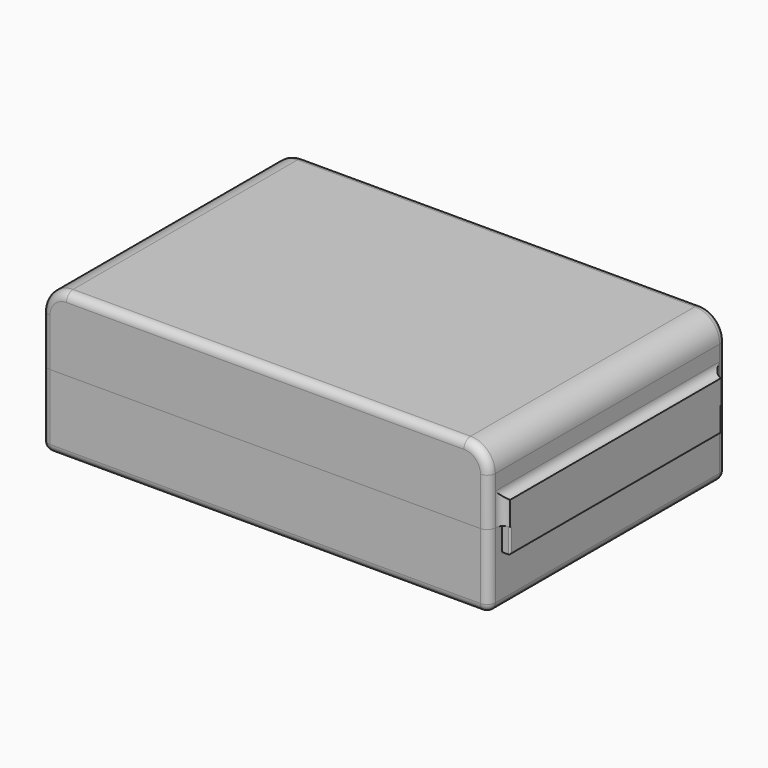
from build123d import *

# Parameters (mm, degrees)
F0_W         = 68.834
F0_H         = 45.72
F1_DEPTH     = 5.08
F2_W         = 68.834
F2_H         = 45.72
F2_W_2       = 58.674
F2_H_2       = 35.56
F3_DEPTH     = 6.35
F4_W         = 68.834
F4_H         = 45.72
F4_W_2       = 58.674
F4_H_2       = 35.56
F5_DEPTH     = 6.35
F6_W         = 68.834
F6_H         = 45.72
F7_DEPTH     = 4.826
F8_W         = 40.64
F8_H         = 3.81
F8_H_2       = 3.683
F9_DEPTH     = 1.27
F10_R        = 3.81
F11_R        = 1.26999
F11_2_R      = 1.26999
F12_T1_DEPTH = 4.4450001001
F12_T3_DEPTH = 41.91


# Not quite as in the source:
# - a fillet or chamfer that OpenCascade refuses, or shapes differently, is made with other operations: its cross-section is extruded or revolved along the edge and cut away or added
# - a fillet or chamfer is up to 0.001 mm smaller than in the source, because OpenCascade refuses the exact size
# - a feature names something its author has since deleted; it is built from what else it names


with BuildPart() as f1:
    # F0 (on Top) → F1 (new body)
    with BuildSketch(Plane.XY):
        with Locations((34.417, 22.86)):
            Rectangle(F0_W, F0_H)
    extrude(amount=F1_DEPTH)

    # F2 (on face) → F3 (join)
    with BuildSketch(Plane.XY.offset(5.08)):
        with Locations((34.417, 22.86)):
            Rectangle(F2_W, F2_H)
        with Locations((34.417, 22.86)):
            Rectangle(F2_W_2, F2_H_2, mode=Mode.SUBTRACT)
    extrude(amount=F3_DEPTH)

    # F11 (radius 1.27 in the source; OpenCascade refuses exactly that, so slightly less here)
    f11_edges = [f1.edges().sort_by_distance(p)[0] for p in [
        (68.834, 0, 5.715),
        (0, 0, 5.715),
        (34.417, 0, 0),
        (68.834, 22.86, 0),
        (68.834, 45.72, 5.715),
        (34.417, 45.72, 0),
        (0, 45.72, 5.715),
        (0, 22.86, 0),
    ]]
    fillet(f11_edges, radius=F11_R)


with BuildPart() as f5:
    # F4 (on face) → F5 (new body)
    with BuildSketch(Plane.XY.offset(11.43)):
        with Locations((34.417, 22.86)):
            Rectangle(F4_W, F4_H)
        with Locations((34.417, 22.86)):
            Rectangle(F4_W_2, F4_H_2, mode=Mode.SUBTRACT)
    extrude(amount=F5_DEPTH)

    # F6 (on face) → F7 (join)
    with BuildSketch(Plane.XY.offset(17.78)):
        with Locations((34.417, 22.86)):
            Rectangle(F6_W, F6_H)
    extrude(amount=F7_DEPTH)

    # F8 (on face) → F9 (join)
    with BuildSketch(Plane.YZ.offset(68.834)):
        with Locations((22.86, 9.525)):
            Rectangle(F8_W, F8_H)
        with Locations((22.86, 13.2715)):
            Rectangle(F8_W, F8_H_2)
    extrude(amount=F9_DEPTH)

    # F10
    f10_edges = [f5.edges().sort_by_distance(p)[0] for p in [
        (68.834, 22.86, 22.606),
        (0, 22.86, 22.606),
    ]]
    fillet(f10_edges, radius=F10_R)

    # F11#2 (radius 1.27 in the source; OpenCascade refuses exactly that, so slightly less here)
    f11_2_edges = [f5.edges().sort_by_distance(p)[0] for p in [
        (34.417, 0, 22.606),
        (34.417, 45.72, 22.606),
        (68.834, 22.86, 15.113),
        (68.834, 2.54, 13.2715),
        (68.834, 43.18, 13.2715),
        (68.834, 45.72, 15.113),
        (67.718077, 45.72, 21.490077),
        (0, 45.72, 15.113),
        (1.115923, 45.72, 21.490077),
        (68.834, 0, 15.113),
        (67.718077, 0, 21.490077),
        (0, 0, 15.113),
        (1.115923, 0, 21.490077),
    ]]
    fillet(f11_2_edges, radius=F11_2_R)

    # F12: fillet of radius 0.254 on 7 edges, made by hand

    # F12_s2 → F12_t1 (cut)
    with BuildSketch(Plane.XY.offset(6.985)):
        with BuildLine():
            ThreePointArc((69.85, 2.54), (70.0296051224, 2.6143948776), (70.104, 2.794))
            Line((70.104, 2.794), (70.104, 2.54))
            Line((70.104, 2.54), (69.85, 2.54))
        make_face()
        with BuildLine():
            ThreePointArc((69.85, 43.18), (70.0296051224, 43.1056051224), (70.104, 42.926))
            Line((70.104, 42.926), (70.104, 43.18))
            Line((70.104, 43.18), (69.85, 43.18))
        make_face()
    extrude(amount=F12_T1_DEPTH, mode=Mode.SUBTRACT)

    # F12_s4 → F12_t3 (cut)
    with BuildSketch(Plane.XZ.offset(-43.815)):
        with BuildLine():
            ThreePointArc((70.104, 7.874), (70.0296051224, 7.6943948776), (69.85, 7.62))
            Line((69.85, 7.62), (70.104, 7.62))
            Line((70.104, 7.62), (70.104, 7.874))
        make_face()
    extrude(amount=F12_T3_DEPTH, mode=Mode.SUBTRACT)


solid = Compound([f1.part, f5.part])
